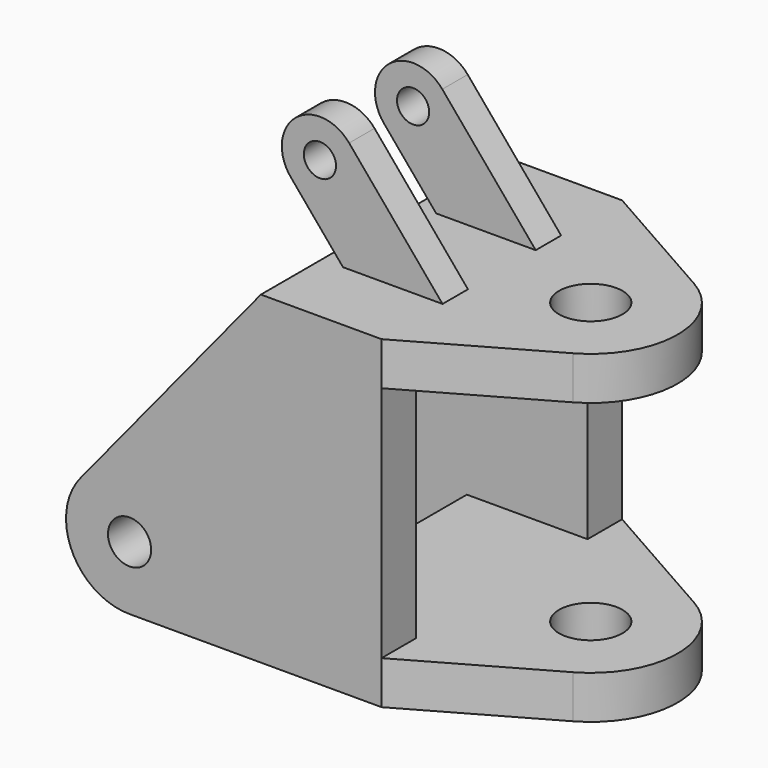
from build123d import *

# Parameters (mm, degrees)
F1_R      = 51
F2_DEPTH  = 102
F4_W      = 285
F4_H      = 102
F4_R      = 75
F5_DEPTH  = 102
F9_R      = 38
F10_DEPTH = 75


# Not quite as in the source:
# - a pattern or mirror of a feature is missing from the dataset's text; its kind, count and spacing are read off the source's solid


with BuildPart() as f2:
    # F1 (on offset) → F2 (new body)
    with BuildSketch(Plane.XZ.offset(253)):
        with BuildLine():
            Line((0, -382.5), (0, 382.5))
            Line((0, 382.5), (-285, 382.5))
            Line((-285, 382.5), (-711.024961042, -137.4305074422))
            ThreePointArc((-711.024961042, -137.4305074422), (-730.5736402913, -296.6855751565), (-595, -382.5))
            Line((-595, -382.5), (0, -382.5))
        make_face()
        with Locations((-595, -232.5)):
            Circle(F1_R, mode=Mode.SUBTRACT)
    extrude(amount=F2_DEPTH)


with BuildPart() as f3_1:
    # F3: instance of F2
    add(f2.part.mirror(Plane.XZ))


with BuildPart() as f5:
    # F4 (on face) → F5 (new body)
    with BuildSketch(Plane.XY.offset(382.5)):
        with Locations((-142.5, -304)):
            Rectangle(F4_W, F4_H)
        with BuildLine():
            Line((311.2296497268, 178.2626096976), (0, 355))
            Line((0, 355), (-285, 355))
            Line((-285, 355), (-285, -253))
            Line((-285, -253), (0, -253))
            Line((0, -253), (0, -355))
            Line((0, -355), (311.2296497268, -178.2626096976))
            ThreePointArc((311.2296497268, -178.2626096976), (415, 0), (311.2296497268, 178.2626096976))
        make_face()
        with Locations((210, 0)):
            Circle(F4_R, mode=Mode.SUBTRACT)
    extrude(amount=-F5_DEPTH)


with BuildPart() as f6_1:
    # F6: instance of F5
    add(f5.part.mirror(Plane.XY))

    # F7: union F2, F3_1, F5
    add(f2.part)
    add(f3_1.part)
    add(f5.part)

    # F9 (on offset) → F10 (join)
    with BuildSketch(Plane.XZ.offset(100)):
        with BuildLine():
            Line((-234.9733120798, 382.5), (0, 382.5))
            Line((0, 382.5), (-220.5580805505, 645.3508848718))
            ThreePointArc((-220.5580805505, 645.3508848718), (-347.352965303, 656.4439998807), (-358.446080312, 529.6491151282))
            Line((-358.446080312, 529.6491151282), (-234.9733120798, 382.5))
        make_face()
        with Locations((-289.5020804312, 587.5)):
            Circle(F9_R, mode=Mode.SUBTRACT)
    f10 = extrude(amount=F10_DEPTH)

    # F10_copies: F10 across plane
    add(f10.mirror(Plane.ZX))


solid = f6_1.part
